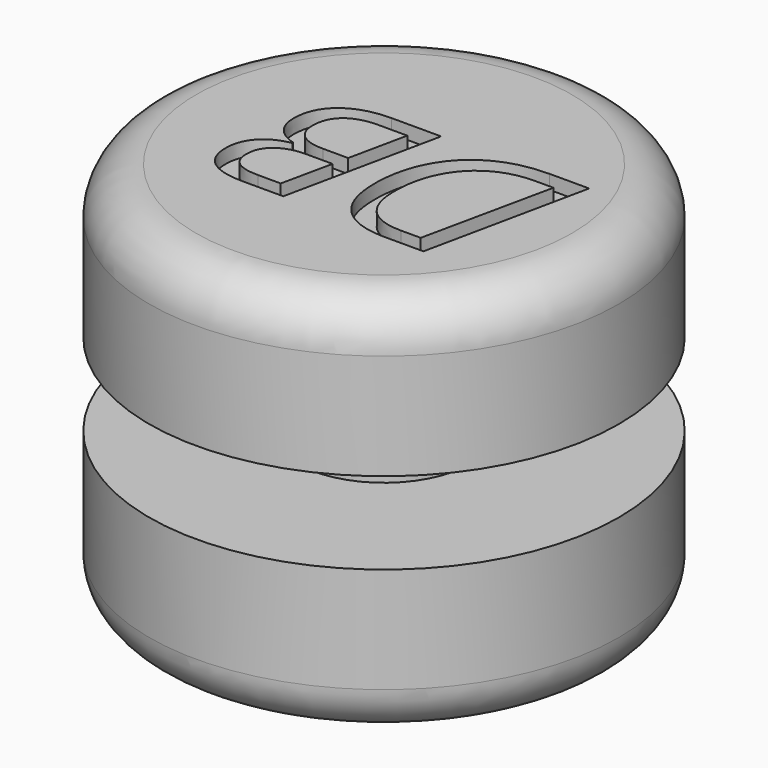
from build123d import *

# Parameters (mm, degrees)
F0_R          = 25.4
F1_DEPTH      = 16.51
F2_R          = 5.08
F4_R          = 9.525
F5_DEPTH      = 8.89
F6_R          = 25.4
F6_R_2        = 9.525
F7_DEPTH      = 12.7
F8_R          = 25.4
F8_R_2        = 9.525
F9_DEPTH      = 3.81
F10_R         = 5.08
F11_R         = 9.525
F12_DEPTH     = 16.51
F13_TEXT_SIZE = 24.8229423608
F14_DEPTH     = 1.524
F15_TEXT_SIZE = 23.6436174924
F16_DEPTH     = 1.524


# Not quite as in the source:
# - Text() gives the source's letters only with a copy of the font that has no kerning and outlines rounded to 1/6400 em; it was checked with that copy


with BuildPart() as f1:
    # F0 (on Top) → F1 (new body)
    with BuildSketch(Plane.XY):
        Circle(F0_R)
    extrude(amount=F1_DEPTH)

    # F2
    f2_edges = [f1.edges().sort_by_distance(p)[0] for p in [
        (-25.4, 0, 16.51),
    ]]
    fillet(f2_edges, radius=F2_R)

    # F4 (on face) → F5 (join)
    with BuildSketch(Plane(origin=(0, 0, 0), x_dir=(1, 0, 0), z_dir=(0, 0, -1))):
        Circle(F4_R)
    extrude(amount=F5_DEPTH)

    # F13 (on face) → F14 (cut)
    with BuildSketch(Plane.XY.offset(16.51)):
        with Locations(Location((17.3683024831, 7.3252691496), (0, 0, -180))):
            Text('D', F13_TEXT_SIZE, font='Open Sans', font_style=FontStyle.ITALIC, text_align=(TextAlign.LEFT, TextAlign.BOTTOM))
    extrude(amount=-F14_DEPTH, mode=Mode.SUBTRACT)

    # F15 (on face) → F16 (cut)
    with BuildSketch(Plane.XY.offset(16.51)):
        with Locations(Location((1.6096126687, 6.9512235932), (0, 0, -180))):
            Text('B', F15_TEXT_SIZE, font='Open Sans', font_style=FontStyle.ITALIC, text_align=(TextAlign.LEFT, TextAlign.BOTTOM))
    extrude(amount=-F16_DEPTH, mode=Mode.SUBTRACT)


with BuildPart() as f7:
    # F6 (on face) → F7 (new body)
    with BuildSketch(Plane(origin=(0, 0, -8.89), x_dir=(1, 0, 0), z_dir=(0, 0, -1))):
        Circle(F6_R)
        Circle(F6_R_2, mode=Mode.SUBTRACT)
    extrude(amount=F7_DEPTH)

    # F8 (on face) → F9 (join)
    with BuildSketch(Plane(origin=(0, 0, -21.59), x_dir=(1, 0, 0), z_dir=(0, 0, -1))):
        Circle(F8_R)
        Circle(F8_R_2, mode=Mode.SUBTRACT)
    extrude(amount=F9_DEPTH)

    # F10
    f10_edges = [f7.edges().sort_by_distance(p)[0] for p in [
        (-25.4, 0, -25.4),
    ]]
    fillet(f10_edges, radius=F10_R)


with BuildPart() as f12:
    # F11 (on face) → F12 (new body)
    with BuildSketch(Plane(origin=(0, 0, -8.89), x_dir=(1, 0, 0), z_dir=(0, 0, -1))):
        Circle(F11_R)
    extrude(amount=F12_DEPTH)


solid = Compound([f1.part, f7.part, f12.part])
